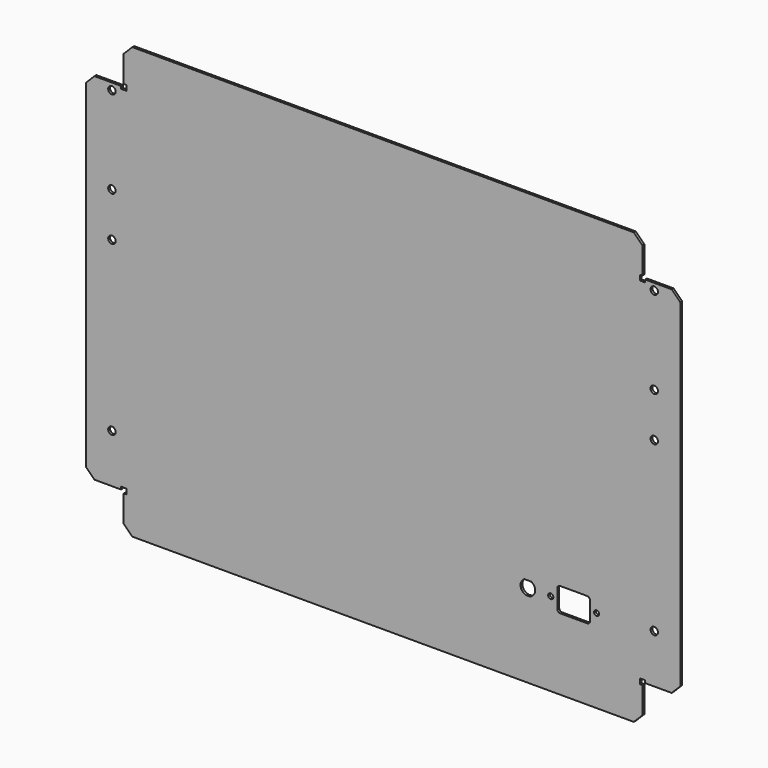
from build123d import *

# Parameters (mm, degrees)
F0_R     = 2.25
F1_DEPTH = 1
F2_SIZE  = 7.5
F3_R     = 3.25
F4_DEPTH = 2


# Not quite as in the source:
# - a feature names something its author has since deleted; it is built from what else it names


with BuildPart() as f1:
    # F0 (on Front) → F1 (new body, symmetric)
    with BuildSketch(Plane.XZ):
        Polygon((226.3, 155), (226.3, 188), (-226.3, 188), (-226.3, 155), (-259.3, 155), (-259.3, -155), (-226.3, -155), (-226.3, -188), (226.3, -188), (226.3, -155), (259.3, -155), (259.3, 155), align=None)
        with BuildLine():
            ThreePointArc((129.1982753492, -109.35), (126.3, -121.35), (123.4017246508, -109.35))
            Line((123.4017246508, -109.35), (129.1982753492, -109.35))
        make_face(mode=Mode.SUBTRACT)
        with Locations((146.3, -115)):
            Circle(F0_R, mode=Mode.SUBTRACT)
        with BuildLine():
            Line((154.55, -104.5), (178.05, -104.5))
            ThreePointArc((178.05, -104.5), (179.817766953, -105.232233047), (180.55, -107))
            Line((180.55, -107), (180.55, -123))
            ThreePointArc((180.55, -123), (179.817766953, -124.767766953), (178.05, -125.5))
            Line((178.05, -125.5), (154.55, -125.5))
            ThreePointArc((154.55, -125.5), (152.782233047, -124.767766953), (152.05, -123))
            Line((152.05, -123), (152.05, -107))
            ThreePointArc((152.05, -107), (152.782233047, -105.232233047), (154.55, -104.5))
        make_face(mode=Mode.SUBTRACT)
        with Locations((186.3, -115)):
            Circle(F0_R, mode=Mode.SUBTRACT)
    extrude(amount=F1_DEPTH, both=True)

    # F2
    f2_edges = [f1.edges().sort_by_distance(p)[0] for p in [
        (226.3, 0, 188),
        (259.3, 0, 155),
        (259.3, 0, -155),
        (226.3, 0, -188),
        (-226.3, 0, 188),
        (-259.3, 0, 155),
        (-259.3, 0, -155),
        (-226.3, 0, -188),
    ]]
    chamfer(f2_edges, length=F2_SIZE)

    # F3 (on face) → F4 (cut, through all)
    with BuildSketch(Plane.XZ.offset(1)):
        Polygon((-228.55, -152.75), (-228.55, -155), (-226.3, -155), (-226.3, -157.25), (-224.05, -157.25), (-224.05, -152.75), align=None)
        Polygon((226.3, -155), (228.55, -155), (228.55, -152.75), (224.05, -152.75), (224.05, -157.25), (226.3, -157.25), align=None)
        with Locations((-236.6, 149.1)):
            Circle(F3_R)
        with Locations((-236.6, 72.9)):
            Circle(F3_R)
        with Locations((-236.6, 34.3)):
            Circle(F3_R)
        with Locations((-236.6, -112.4)):
            Circle(F3_R)
        with Locations((236.6, -112.4)):
            Circle(F3_R)
        with Locations((236.6, 34.3)):
            Circle(F3_R)
        with Locations((236.6, 72.9)):
            Circle(F3_R)
        with Locations((236.6, 149.1)):
            Circle(F3_R)
        Polygon((226.3, 155), (226.3, 157.25), (224.05, 157.25), (224.05, 152.75), (228.55, 152.75), (228.55, 155), align=None)
        Polygon((-224.05, 152.75), (-224.05, 157.25), (-226.3, 157.25), (-226.3, 155), (-228.55, 155), (-228.55, 152.75), align=None)
    extrude(amount=-F4_DEPTH, mode=Mode.SUBTRACT)


solid = f1.part
